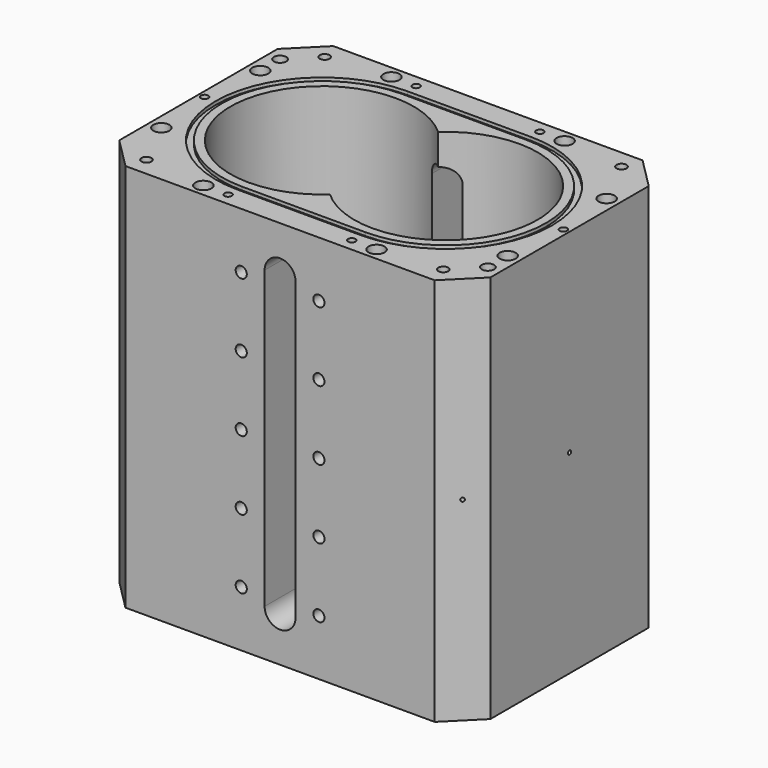
from build123d import *

# Parameters (mm, degrees)
F0_W          = 300
F0_H          = 210
F1_DEPTH      = 157.14
F1_DEPTH_BACK = 157.14
F3_DEPTH      = 105
F3_DEPTH_BACK = 105
F4_R          = 4.5
F5_DEPTH      = 21
F6_R          = 6.5
F6_R_2        = 4.25
F7_DEPTH      = 20
F6_R_3        = 3
F8_DEPTH      = 10
F6_R_4        = 5
F9_DEPTH      = 40
F6_R_5        = 4
F10_DEPTH     = 16
F11_SIZE      = 25
F12_R         = 1.5875
F12_R_2       = 1.5
F13_DEPTH     = 10
F14_DEPTH     = 40
F15_R         = 1.5
F16_DEPTH     = 70
F17_R         = 1.5
F18_DEPTH     = 70
F20_DEPTH     = 2.7
F22_DEPTH     = 2.7
F23_R         = 4.5
F24_DEPTH     = 21


# Not quite as in the source:
# - a feature names something its author has since deleted; it is built from what else it names


with BuildPart() as f1:
    # F0 (on Top) → F1 (new body, two sides)
    with BuildSketch(Plane.XY) as f1_sk:
        Rectangle(F0_W, F0_H)
        with BuildLine():
            ThreePointArc((-50, -86), (-136, 0), (-50, 86))
            Line((-50, 86), (50, 86))
            ThreePointArc((50, 86), (136, 0), (50, -86))
            Line((50, -86), (-50, -86))
        make_face(mode=Mode.SUBTRACT)
        with BuildLine():
            Line((50, 86), (-50, 86))
            ThreePointArc((-50, 86), (-136, 0), (-50, -86))
            Line((-50, -86), (50, -86))
            ThreePointArc((50, -86), (136, 0), (50, 86))
        make_face()
        with BuildLine():
            ThreePointArc((-50, -81), (-131, 0), (-50, 81))
            Line((-50, 81), (50, 81))
            ThreePointArc((50, 81), (131, 0), (50, -81))
            Line((50, -81), (-50, -81))
        make_face(mode=Mode.SUBTRACT)
        with BuildLine():
            Line((50, 81), (-50, 81))
            ThreePointArc((-50, 81), (-131, 0), (-50, -81))
            Line((-50, -81), (50, -81))
            ThreePointArc((50, -81), (131, 0), (50, 81))
        make_face()
        with BuildLine():
            ThreePointArc((0, -54.6611964743), (-124.08, 0), (0, 54.6611964743))
            ThreePointArc((0, 54.6611964743), (124.08, 0), (0, -54.6611964743))
        make_face(mode=Mode.SUBTRACT)
    extrude(amount=F1_DEPTH)
    extrude(f1_sk.sketch, amount=-F1_DEPTH_BACK)

    # F2 (on Front) → F3 (cut, two sides)
    with BuildSketch(Plane.XZ) as f3_sk:
        with BuildLine():
            ThreePointArc((12.5, 119.64), (0, 132.14), (-12.5, 119.64))
            Line((-12.5, 119.64), (-12.5, -119.64))
            ThreePointArc((-12.5, -119.64), (0, -132.14), (12.5, -119.64))
            Line((12.5, -119.64), (12.5, 119.64))
        make_face()
    extrude(amount=-F3_DEPTH, mode=Mode.SUBTRACT)
    extrude(f3_sk.sketch, amount=F3_DEPTH_BACK, mode=Mode.SUBTRACT)

    # F4 (on face) → F5 (cut)
    with BuildSketch(Plane.XZ.offset(105)):
        with Locations((-31.4, 112)):
            Circle(F4_R)
        with Locations((-31.4, 56)):
            Circle(F4_R)
        with Locations((-31.4, 0)):
            Circle(F4_R)
        with Locations((-31.4, -56)):
            Circle(F4_R)
        with Locations((-31.4, -112)):
            Circle(F4_R)
        with Locations((31.4, -112)):
            Circle(F4_R)
        with Locations((31.4, -56)):
            Circle(F4_R)
        with Locations((31.4, 0)):
            Circle(F4_R)
        with Locations((31.4, 56)):
            Circle(F4_R)
        with Locations((31.4, 112)):
            Circle(F4_R)
    extrude(amount=-F5_DEPTH, mode=Mode.SUBTRACT)

    # F6 (on face) → F7 (cut)
    with BuildSketch(Plane.XY.offset(157.14)):
        with Locations((140, 50)):
            Circle(F6_R)
        with Locations((140, 50)):
            Circle(F6_R_2, mode=Mode.SUBTRACT)
        with Locations((140, -50)):
            Circle(F6_R)
        with Locations((140, -50)):
            Circle(F6_R_2, mode=Mode.SUBTRACT)
        with Locations((70, -95)):
            Circle(F6_R)
        with Locations((70, -95)):
            Circle(F6_R_2, mode=Mode.SUBTRACT)
        with Locations((-70, -95)):
            Circle(F6_R)
        with Locations((-70, -95)):
            Circle(F6_R_2, mode=Mode.SUBTRACT)
        with Locations((-140, -50)):
            Circle(F6_R)
        with Locations((-140, -50)):
            Circle(F6_R_2, mode=Mode.SUBTRACT)
        with Locations((-140, 50)):
            Circle(F6_R)
        with Locations((-140, 50)):
            Circle(F6_R_2, mode=Mode.SUBTRACT)
        with Locations((-70, 95)):
            Circle(F6_R)
        with Locations((-70, 95)):
            Circle(F6_R_2, mode=Mode.SUBTRACT)
        with Locations((70, 95)):
            Circle(F6_R)
        with Locations((70, 95)):
            Circle(F6_R_2, mode=Mode.SUBTRACT)
    extrude(amount=-F7_DEPTH, mode=Mode.SUBTRACT)

    # F6 (on face) → F8 (cut)
    with BuildSketch(Plane.XY.offset(157.14)):
        with Locations((-50, 95)):
            Circle(F6_R_3)
        with Locations((-145, 0)):
            Circle(F6_R_3)
        with Locations((50, 95)):
            Circle(F6_R_3)
        with Locations((145, 0)):
            Circle(F6_R_3)
        with Locations((-50, -95)):
            Circle(F6_R_3)
        with Locations((50, -95)):
            Circle(F6_R_3)
    extrude(amount=-F8_DEPTH, mode=Mode.SUBTRACT)

    # F6 (on face) → F9 (cut)
    with BuildSketch(Plane.XY.offset(157.14)):
        with Locations((-70, 95)):
            Circle(F6_R_2)
        with Locations((-140, 50)):
            Circle(F6_R_2)
        with Locations((-140, -50)):
            Circle(F6_R_2)
        with Locations((-70, -95)):
            Circle(F6_R_2)
        with Locations((70, -95)):
            Circle(F6_R_2)
        with Locations((140, -50)):
            Circle(F6_R_2)
        with Locations((140, 50)):
            Circle(F6_R_2)
        with Locations((70, 95)):
            Circle(F6_R_2)
        with Locations((-140, 70)):
            Circle(F6_R_4)
        with Locations((140, -70)):
            Circle(F6_R_4)
    extrude(amount=-F9_DEPTH, mode=Mode.SUBTRACT)

    # F6 (on face) → F10 (cut)
    with BuildSketch(Plane.XY.offset(157.14)):
        with Locations((-120, 90)):
            Circle(F6_R_5)
        with Locations((-120, -90)):
            Circle(F6_R_5)
        with Locations((120, -90)):
            Circle(F6_R_5)
        with Locations((120, 90)):
            Circle(F6_R_5)
    extrude(amount=-F10_DEPTH, mode=Mode.SUBTRACT)

    # F11
    f11_edges = [f1.edges().sort_by_distance(p)[0] for p in [
        (-150, 105, 0),
        (-150, -105, 0),
        (150, 105, 0),
        (150, -105, 0),
    ]]
    chamfer(f11_edges, length=F11_SIZE)

    # F12 (on face) → F13 (cut)
    with BuildSketch(Plane.YZ.offset(150)):
        Circle(F12_R)
        Circle(F12_R_2, mode=Mode.SUBTRACT)
    extrude(amount=-F13_DEPTH, mode=Mode.SUBTRACT)

    # F14 (cut): a face of the model
    f14_faces = [f1.faces().sort_by_distance(p)[0] for p in [
        (150, 0, 0),
    ]]
    extrude(f14_faces, amount=-F14_DEPTH, mode=Mode.SUBTRACT)

    # F15 (on face) → F16 (cut)
    with BuildSketch(Plane(origin=(115, -115, 0), x_dir=(0.7071067812, 0.7071067812, 0), z_dir=(0.7071067812, -0.7071067812, 0))):
        with Locations((31.8221356237, 0)):
            Circle(F15_R)
    extrude(amount=-F16_DEPTH, mode=Mode.SUBTRACT)

    # F17 (on face) → F18 (cut)
    with BuildSketch(Plane(origin=(115, 115, 0), x_dir=(-0.7071067812, 0.7071067812, 0), z_dir=(0.7071067812, 0.7071067812, 0))):
        with Locations((-31.8174746831, 0)):
            Circle(F17_R)
    extrude(amount=-F18_DEPTH, mode=Mode.SUBTRACT)

    # F19 (on face) → F20 (cut)
    with BuildSketch(Plane.XY.offset(157.14)):
        with BuildLine():
            Line((-50, -86), (50, -86))
            ThreePointArc((50, -86), (136, 0), (50, 86))
            Line((50, 86), (-50, 86))
            ThreePointArc((-50, 86), (-136, 0), (-50, -86))
        make_face()
        with BuildLine():
            ThreePointArc((50, 81), (131, 0), (50, -81))
            Line((50, -81), (-50, -81))
            ThreePointArc((-50, -81), (-131, 0), (-50, 81))
            Line((-50, 81), (50, 81))
        make_face(mode=Mode.SUBTRACT)
    extrude(amount=-F20_DEPTH, mode=Mode.SUBTRACT)

    # F21 (on face) → F22 (cut)
    with BuildSketch(Plane(origin=(0, 0, -157.14), x_dir=(1, 0, 0), z_dir=(0, 0, -1))):
        with BuildLine():
            Line((50, 86), (-50, 86))
            ThreePointArc((-50, 86), (-136, 0), (-50, -86))
            Line((-50, -86), (50, -86))
            ThreePointArc((50, -86), (136, 0), (50, 86))
        make_face()
        with BuildLine():
            ThreePointArc((-50, -81), (-131, 0), (-50, 81))
            Line((-50, 81), (50, 81))
            ThreePointArc((50, 81), (131, 0), (50, -81))
            Line((50, -81), (-50, -81))
        make_face(mode=Mode.SUBTRACT)
    extrude(amount=-F22_DEPTH, mode=Mode.SUBTRACT)

    # F23 (on face) → F24 (cut)
    with BuildSketch(Plane(origin=(0, 105, 0), x_dir=(-1, 0, 0), z_dir=(0, 1, 0))):
        with Locations((32.3209376876, -110.7883939175)):
            Circle(F23_R)
        with Locations((-30.4790623124, -110.7883939175)):
            Circle(F23_R)
        with Locations((32.3209376876, -54.7883939175)):
            Circle(F23_R)
        with Locations((32.3209376876, 1.2116060825)):
            Circle(F23_R)
        with Locations((32.3209376876, 57.2116060825)):
            Circle(F23_R)
        with Locations((32.3209376876, 113.2116060825)):
            Circle(F23_R)
        with Locations((-30.4790623124, 113.2116060825)):
            Circle(F23_R)
        with Locations((-30.4790623124, 57.2116060825)):
            Circle(F23_R)
        with Locations((-30.4790623124, 1.2116060825)):
            Circle(F23_R)
        with Locations((-30.4790623124, -54.7883939175)):
            Circle(F23_R)
    extrude(amount=-F24_DEPTH, mode=Mode.SUBTRACT)


solid = f1.part
